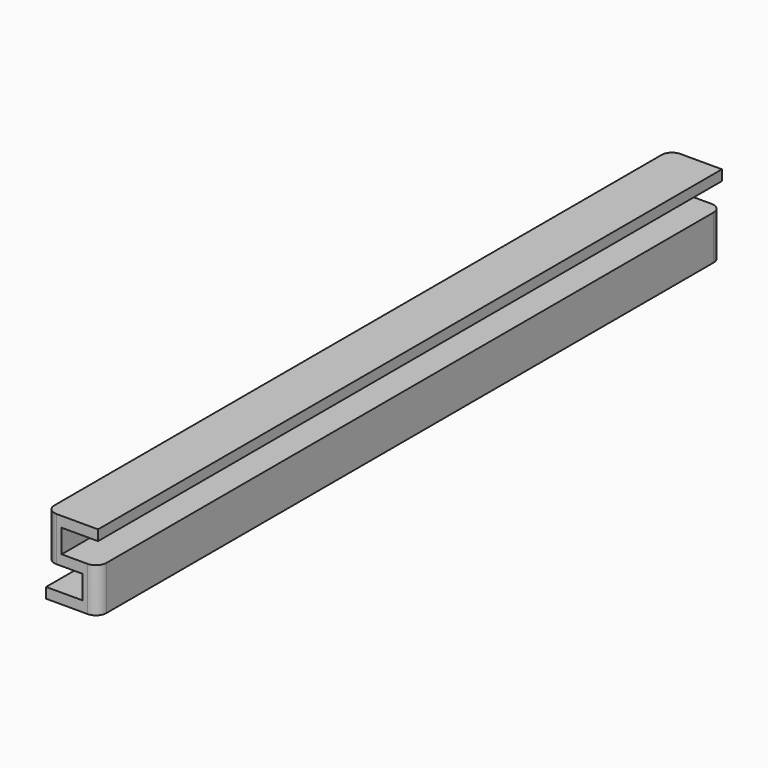
from build123d import *

# Parameters (mm, degrees)
F0_W     = 10
F0_H     = 150
F1_DEPTH = 2
F2_W     = 3
F2_H     = 150
F3_DEPTH = 4.5
F4_W     = 3
F4_H     = 150
F4_W_2   = 7
F5_DEPTH = 2
F6_W     = 3
F6_H     = 150
F7_DEPTH = 4.5
F8_W     = 3
F8_H     = 150
F8_W_2   = 7
F9_DEPTH = 2
F10_R    = 2


# Not quite as in the source:
# - a feature names something its author has since deleted; it is built from what else it names


with BuildPart() as f1:
    # F0 (on Top) → F1 (new body)
    with BuildSketch(Plane.XY):
        Rectangle(F0_W, F0_H)
    extrude(amount=F1_DEPTH)

    # F2 (on face) → F3 (join)
    with BuildSketch(Plane.XY.offset(2)):
        with Locations((3.5, 0)):
            Rectangle(F2_W, F2_H)
    extrude(amount=F3_DEPTH)

    # F4 (on face) → F5 (join)
    with BuildSketch(Plane.XY.offset(6.5)):
        with Locations((3.5, 0)):
            Rectangle(F4_W, F4_H)
        with Locations((-1.5, 0)):
            Rectangle(F4_W_2, F4_H)
    extrude(amount=F5_DEPTH)

    # F6 (on face) → F7 (join)
    with BuildSketch(Plane.XY.offset(8.5)):
        with Locations((-3.5, 0)):
            Rectangle(F6_W, F6_H)
    extrude(amount=F7_DEPTH)

    # F8 (on face) → F9 (join)
    with BuildSketch(Plane.XY.offset(13)):
        with Locations((-3.5, 0)):
            Rectangle(F8_W, F8_H)
        with Locations((1.5, 0)):
            Rectangle(F8_W_2, F8_H)
    extrude(amount=F9_DEPTH)

    # F10
    f10_edges = [f1.edges().sort_by_distance(p)[0] for p in [
        (-5, 75, 10.75),
        (5, 75, 4.25),
        (-5, -75, 10.75),
        (5, -75, 4.25),
    ]]
    fillet(f10_edges, radius=F10_R)


solid = f1.part
